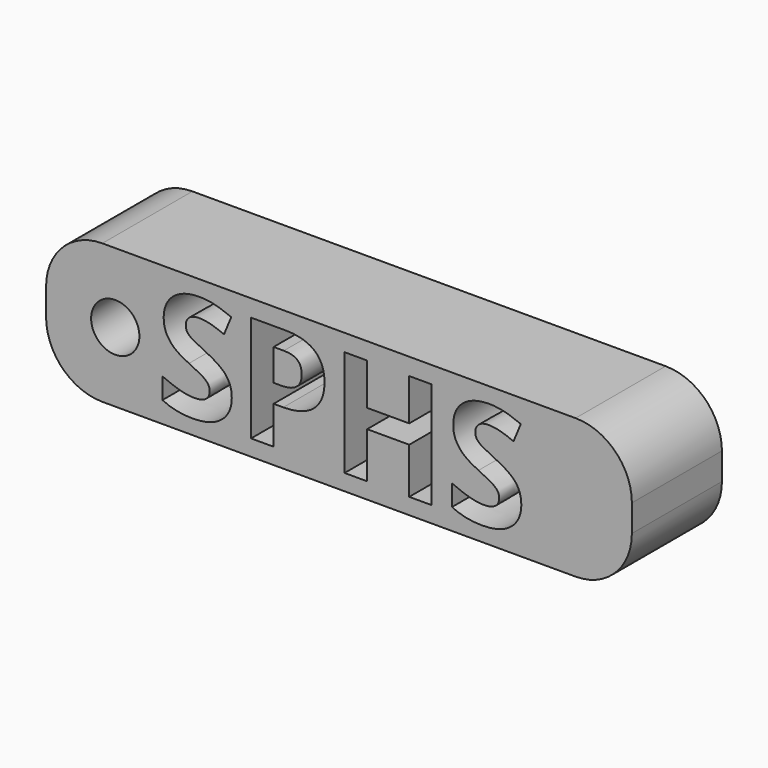
from build123d import *

# Parameters (mm, degrees)
F0_W         = 132.1791261435
F0_H         = 31.4836129546
F1_DEPTH     = 25.4
F2_TEXT_SIZE = 33.6085368569
F3_DEPTH     = 25.4
F4_R         = 12.7
F5_R         = 12.7
F6_R         = 12.7
F7_R         = 12.7
F8_R         = 5.4470328303
F9_DEPTH     = 25.4010001


# Not quite as in the source:
# - Text() gives the source's letters only with a copy of the font that has no kerning and outlines rounded to 1/6400 em; it was checked with that copy


with BuildPart() as f1:
    # F0 (on Front) → F1 (new body)
    with BuildSketch(Plane.XZ):
        Rectangle(F0_W, F0_H)
    extrude(amount=F1_DEPTH)

    # F2 (on face) → F3 (cut)
    with BuildSketch(Plane.XZ.offset(25.4)):
        with Locations((-41.3710251451, -12.0990723372)):
            Text('SPHS', F2_TEXT_SIZE, font='Open Sans', font_style=FontStyle.BOLD, text_align=(TextAlign.LEFT, TextAlign.BOTTOM))
    extrude(amount=-F3_DEPTH, mode=Mode.SUBTRACT)

    # F4
    f4_edges = [f1.edges().sort_by_distance(p)[0] for p in [
        (66.089563, -12.7, 15.741806),
    ]]
    fillet(f4_edges, radius=F4_R)

    # F5
    f5_edges = [f1.edges().sort_by_distance(p)[0] for p in [
        (66.089563, -12.7, -15.741806),
    ]]
    fillet(f5_edges, radius=F5_R)

    # F6
    f6_edges = [f1.edges().sort_by_distance(p)[0] for p in [
        (-66.089563, -12.7, 15.741806),
    ]]
    fillet(f6_edges, radius=F6_R)

    # F7
    f7_edges = [f1.edges().sort_by_distance(p)[0] for p in [
        (-66.089563, -12.7, -15.741806),
    ]]
    fillet(f7_edges, radius=F7_R)

    # F8 (on face) → F9 (cut, through all)
    with BuildSketch(Plane.XZ.offset(25.4)):
        with Locations((-50.4778549075, 0)):
            Circle(F8_R)
    extrude(amount=-F9_DEPTH, mode=Mode.SUBTRACT)


solid = f1.part
